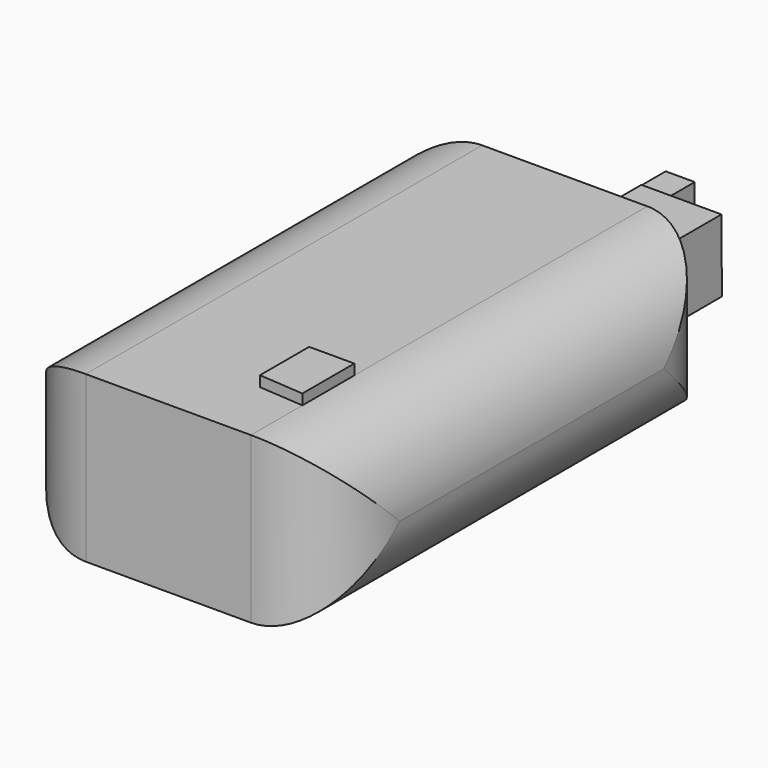
from build123d import *

# Parameters (mm, degrees)
F0_W     = 80
F0_H     = 120
F1_DEPTH = 40
F2_R     = 19.99999
F4_DEPTH = 2.54
F6_DEPTH = 15
F8_DEPTH = 10


# Not quite as in the source:
# - a fillet or chamfer is up to 0.001 mm smaller than in the source, because OpenCascade refuses the exact size


with BuildPart() as f1:
    # F0 (on Top) → F1 (new body)
    with BuildSketch(Plane.XY):
        with Locations((-88.8195456503, -59.9255193707)):
            Rectangle(F0_W, F0_H)
    extrude(amount=F1_DEPTH)

    # F2 (radius 20 in the source; OpenCascade refuses exactly that, so slightly less here)
    f2_edges = [f1.edges().sort_by_distance(p)[0] for p in [
        (-48.819546, -119.925519, 20),
        (-48.819546, 0.074481, 20),
        (-48.819546, -59.925519, 0),
        (-48.819546, -59.925519, 40),
        (-128.819546, 0.074481, 20),
        (-128.819546, -119.925519, 20),
        (-128.819546, -59.925519, 0),
        (-128.819546, -59.925519, 40),
    ]]
    fillet(f2_edges, radius=F2_R)

    # F3 (on face) → F4 (join)
    with BuildSketch(Plane.XY.offset(40)):
        Polygon((-79.7564014792, -103.5247588724), (-68.8195456503, -104.3402352648), (-68.8195456503, -88.6302217841), (-79.7564014792, -88.6302217841), align=None)
    extrude(amount=F4_DEPTH)


with BuildPart() as f6:
    # F5 (on face) → F6 (new body)
    with BuildSketch(Plane(origin=(0, 0.0744806293, 0), x_dir=(-1, 0, 0), z_dir=(0, 1, 0))):
        Polygon((82.2559818625, 34.1151989996), (62.8604739904, 34.1151989996), (62.7438053489, 16.6449602693), (82.2559818625, 16.6449602693), align=None)
    extrude(amount=F6_DEPTH)


with BuildPart() as f8:
    # F7 (on face) → F8 (new body)
    with BuildSketch(Plane(origin=(0, 15.0744806293, 0), x_dir=(-1, 0, 0), z_dir=(0, 1, 0))):
        Polygon((77.3247284815, 32.2467796504), (77.3247284815, 25.3800796345), (84.357063286, 24.1537168622), (84.357063286, 32.2467796504), align=None)
    extrude(amount=F8_DEPTH)


solid = Compound([f1.part, f6.part, f8.part])
